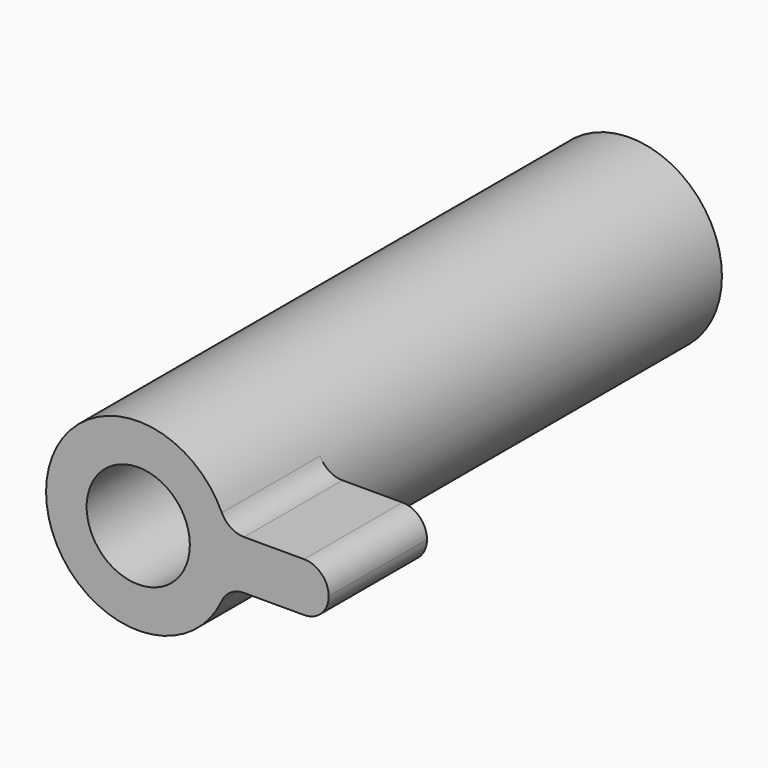
from build123d import *

# Parameters (mm, degrees)
F0_R     = 3.75
F1_DEPTH = 25
F2_W     = 8
F2_H     = 2
F3_DEPTH = 5
F4_R     = 0.99999
F5_R     = 2.1
F6_DEPTH = 15
F7_R     = 3
F7_R_2   = 2.75
F8_DEPTH = 1
F9_R     = 1


# Not quite as in the source:
# - a fillet or chamfer is up to 0.001 mm smaller than in the source, because OpenCascade refuses the exact size


with BuildPart() as f1:
    # F0 (on Front) → F1 (new body)
    with BuildSketch(Plane.XZ):
        Circle(F0_R)
    extrude(amount=F1_DEPTH)

    # F2 (on face) → F3 (join)
    with BuildSketch(Plane.XZ.offset(25)):
        with Locations((3.75, 0)):
            Rectangle(F2_W, F2_H)
    extrude(amount=-F3_DEPTH)

    # F4 (radius 1 in the source; OpenCascade refuses exactly that, so slightly less here)
    f4_edges = [f1.edges().sort_by_distance(p)[0] for p in [
        (3.614208, -22.5, 1),
        (3.614208, -22.5, -1),
        (7.75, -22.5, 1),
        (7.75, -22.5, -1),
    ]]
    fillet(f4_edges, radius=F4_R)

    # F5 (on face) → F6 (cut)
    with BuildSketch(Plane.XZ.offset(25)):
        Circle(F5_R)
    extrude(amount=-F6_DEPTH, mode=Mode.SUBTRACT)

    # F7 (on face) → F8 (cut)
    with BuildSketch(Plane(origin=(0, 0, 0), x_dir=(-1, 0, 0), z_dir=(0, 1, 0))):
        Circle(F7_R)
        Circle(F7_R_2, mode=Mode.SUBTRACT)
        Polygon((1.25, -2.1650635095), (2.5, 0), (1.25, 2.1650635095), (-1.25, 2.1650635095), (-2.5, 0), (-1.25, -2.1650635095), align=None)
        with BuildLine():
            ThreePointArc((1, 1.7320508076), (1.7320508076, 1), (2, 0))
            ThreePointArc((2, 0), (1.7320508076, -1), (1, -1.7320508076))
            ThreePointArc((1, -1.7320508076), (0, -2), (-1, -1.7320508076))
            ThreePointArc((-1, -1.7320508076), (-1.7320508076, -1), (-2, 0))
            ThreePointArc((-2, 0), (-1.7320508076, 1), (-1, 1.7320508076))
            ThreePointArc((-1, 1.7320508076), (0, 2), (1, 1.7320508076))
        make_face(mode=Mode.SUBTRACT)
        with BuildLine():
            Line((-2, 0), (-1, 1.7320508076))
            ThreePointArc((-1, 1.7320508076), (-1.7320508076, 1), (-2, 0))
        make_face()
        with BuildLine():
            Line((-1, 1.7320508076), (1, 1.7320508076))
            ThreePointArc((1, 1.7320508076), (0, 2), (-1, 1.7320508076))
        make_face()
        with BuildLine():
            ThreePointArc((-2, 0), (-1.7320508076, -1), (-1, -1.7320508076))
            Line((-1, -1.7320508076), (-2, 0))
        make_face()
        with BuildLine():
            ThreePointArc((1, -1.7320508076), (1.7320508076, -1), (2, 0))
            Line((2, 0), (1.5, -0.8660254038))
            Line((1.5, -0.8660254038), (1, -1.7320508076))
        make_face()
        with BuildLine():
            Line((1, 1.7320508076), (2, 0))
            ThreePointArc((2, 0), (1.7320508076, 1), (1, 1.7320508076))
        make_face()
        with BuildLine():
            ThreePointArc((-1, -1.7320508076), (0, -2), (1, -1.7320508076))
            Line((1, -1.7320508076), (-1, -1.7320508076))
        make_face()
        Polygon((0.8465453085, -0.7060742072), (0.8991730442, -0.4951797253), (-0.5881552807, 1.095739762), (-0.7212159254, 1.0418686678), align=None)
        Polygon((-0.7212159254, 1.0418686678), (-0.85427657, 0.9879975736), (-0.8180661444, -1.0666475449), (-0.6253293831, -1.2018198644), align=None)
        Polygon((-0.4325926219, -1.3369921838), (0.7939175728, -0.9169686891), (0.8465453085, -0.7060742072), (-0.6253293831, -1.2018198644), align=None)
        Polygon((-0.8180661444, -1.0666475449), (-0.8110177635, -1.4665854405), (-0.4325926219, -1.3369921838), (-0.6253293831, -1.2018198644), align=None)
        Polygon((0.7939175728, -0.9169686891), (1.1723427144, -0.7873754324), (0.8991730442, -0.4951797253), (0.8465453085, -0.7060742072), align=None)
        Polygon((-0.5881552807, 1.095739762), (-0.8613249509, 1.3879354691), (-0.85427657, 0.9879975736), (-0.7212159254, 1.0418686678), align=None)
    extrude(amount=-F8_DEPTH, mode=Mode.SUBTRACT)

    # F9
    f9_edges = [f1.edges().sort_by_distance(p)[0] for p in [
        (-2.1, -10, 0),
    ]]
    fillet(f9_edges, radius=F9_R)


solid = f1.part
